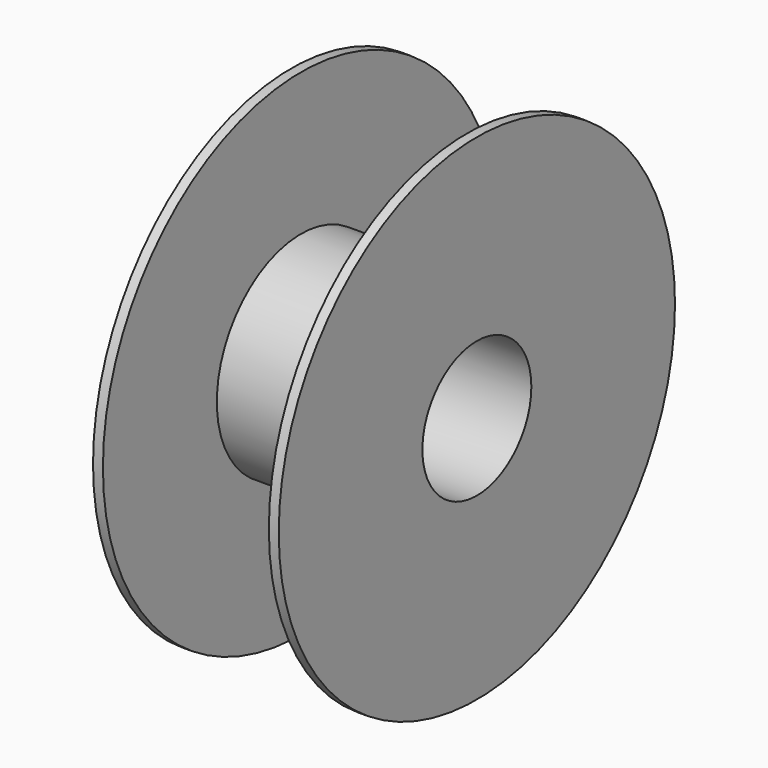
from build123d import *

# Parameters (mm, degrees)
F0_R     = 42.5
F0_R_2   = 27.5
F1_DEPTH = 33.5
F2_R     = 100
F2_R_2   = 42.5
F2_R_3   = 27.5
F3_DEPTH = 4
F4_R     = 100
F4_R_2   = 42.5
F4_R_3   = 27.5
F5_DEPTH = 4


# Not quite as in the source:
# - a feature names something its author has since deleted; it is built from what else it names


with BuildPart() as f1:
    # F0 (on Right) → F1 (new body, symmetric)
    with BuildSketch(Plane.YZ):
        Circle(F0_R)
        Circle(F0_R_2, mode=Mode.SUBTRACT)
    extrude(amount=F1_DEPTH, both=True)

    # F2 (on face) → F3 (join)
    with BuildSketch(Plane.YZ.offset(33.5)):
        Circle(F2_R)
        Circle(F2_R_2, mode=Mode.SUBTRACT)
        Circle(F2_R_2)
        Circle(F2_R_3, mode=Mode.SUBTRACT)
    extrude(amount=F3_DEPTH)

    # F4 (on face) → F5 (join)
    with BuildSketch(Plane(origin=(-33.5, 0, 0), x_dir=(0, -1, 0), z_dir=(-1, 0, 0))):
        Circle(F4_R)
        Circle(F4_R_2, mode=Mode.SUBTRACT)
        Circle(F4_R_2)
        Circle(F4_R_3, mode=Mode.SUBTRACT)
    extrude(amount=F5_DEPTH)


solid = f1.part
